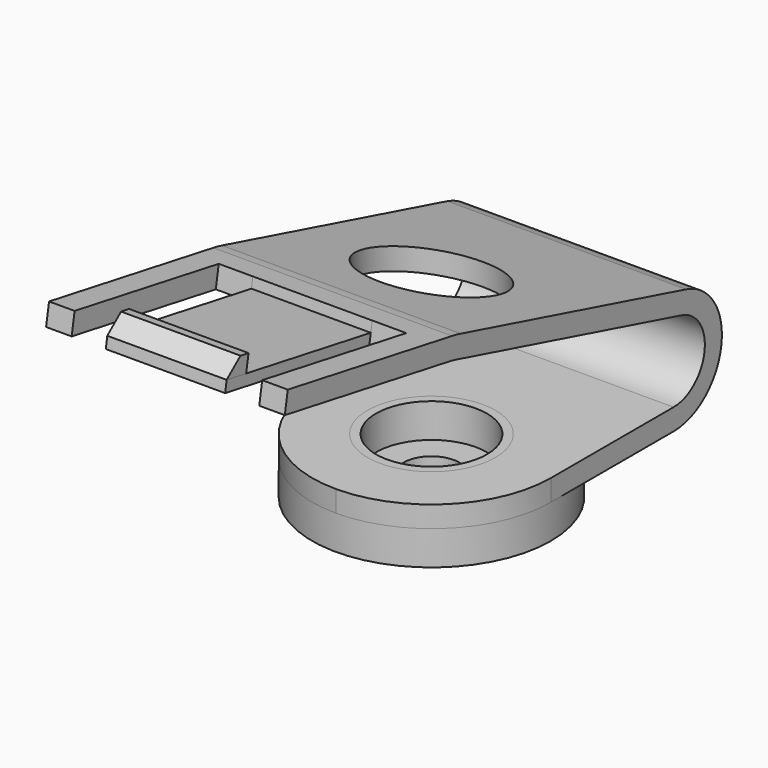
from build123d import *
from build123d import SkipClean  # not in build123d's __all__

# Parameters (mm, degrees)
F1_DEPTH    = 28
F2_T1_DEPTH = 28
F2_T3_DEPTH = 31.2745707181
F3_R        = 14
F4_DEPTH    = 4
F6_DEPTH    = 2.5
F7_R        = 3.25
F8_DEPTH    = 31.3042238242
F9_R        = 7.5
F10_DEPTH   = 24.8042238242
F11_R       = 6.5
F12_DEPTH   = 4
F13_W       = 4
F13_H       = 21.4542382136
F14_DEPTH   = 2.5
F15_W       = 14
F15_H       = 21.4542382136
F16_DEPTH   = 1.2
F18_DEPTH   = 14


# Not quite as in the source:
# - a fillet or chamfer that OpenCascade refuses, or shapes differently, is made with other operations: its cross-section is extruded or revolved along the edge and cut away or added


with BuildPart() as f1:
    # F0 (on Right) → F1 (new body)
    with BuildSketch(Plane.YZ):
        with BuildLine():
            Line((0, 0), (-32, 0))
            Line((-32, 0), (-32, -2.5))
            Line((-32, -2.5), (0, -2.5))
            ThreePointArc((0, -2.5), (7.0205462081, 3.6568537819), (1.8327303277, 11.4209689242))
            Line((1.8327303277, 11.4209689242), (-31.8381916428, 20.4430652746))
            Line((-31.8381916428, 20.4430652746), (-56.5658795558, 24.8032238242))
            Line((-56.5658795558, 24.8032238242), (-57, 22.3412044417))
            Line((-57, 22.3412044417), (-32.3798061747, 18))
            Line((-32.3798061747, 18), (1.1856827149, 9.0061543585))
            ThreePointArc((1.1856827149, 9.0061543585), (4.5419340547, 3.9831692624), (0, 0))
        make_face()
    extrude(amount=F1_DEPTH)

    # F2: fillet of radius 15 on 2 edges, made by hand

    # F2_s2 → F2_t1 (join)
    with BuildSketch(Plane.YZ):
        with BuildLine():
            ThreePointArc((-33.0247707009, 18.1137246476), (-32.3828991568, 17.9860484592), (-31.7472076894, 17.8304957467))
            Line((-31.7472076894, 17.8304957467), (-32.3798061747, 18))
            Line((-32.3798061747, 18), (-33.0247707009, 18.1137246476))
        make_face()
    extrude(amount=F2_T1_DEPTH)

    # F2_s4 → F2_t3 (cut)
    with BuildSketch(Plane.YZ.offset(-1.6372853591)):
        with BuildLine():
            ThreePointArc((-31.2055931575, 20.2735610213), (-31.841284625, 20.4291137338), (-32.483156169, 20.5567899222))
            Line((-32.483156169, 20.5567899222), (-31.8381916428, 20.4430652746))
            Line((-31.8381916428, 20.4430652746), (-31.2055931575, 20.2735610213))
        make_face()
    extrude(amount=F2_T3_DEPTH, mode=Mode.SUBTRACT)

    # F3 (on face) → F4 (join)
    with BuildSketch(Plane(origin=(0, 0, -2.5), x_dir=(1, 0, 0), z_dir=(0, 0, -1))):
        with Locations((14, 18)):
            Circle(F3_R)
    extrude(amount=F4_DEPTH)

    # F5 (on face) → F6 (cut, through all)
    with BuildSketch(Plane(origin=(0, 0, -2.5), x_dir=(1, 0, 0), z_dir=(0, 0, -1))):
        with BuildLine():
            ThreePointArc((0, 18), (4.1005050634, 27.8994949366), (14, 32))
            Line((14, 32), (0, 32))
            Line((0, 32), (0, 18))
        make_face()
        with BuildLine():
            Line((28, 18), (28, 32))
            Line((28, 32), (14, 32))
            ThreePointArc((14, 32), (23.8994949366, 27.8994949366), (28, 18))
        make_face()
    with SkipClean():  # cleaning this boolean's faces spoils the solid; the shape is the same uncleaned
        extrude(amount=-F6_DEPTH, mode=Mode.SUBTRACT)

    # F7 (on face) → F8 (cut, through all)
    with BuildSketch(Plane(origin=(0, 0, -6.5), x_dir=(1, 0, 0), z_dir=(0, 0, -1))):
        with Locations((14, 18)):
            Circle(F7_R)
    with SkipClean():  # cleaning this boolean's faces spoils the solid; the shape is the same uncleaned
        extrude(amount=-F8_DEPTH, mode=Mode.SUBTRACT)

    # F9 (on face) → F10 (cut, through all)
    with BuildSketch(Plane.XY):
        with Locations((14, -18)):
            Circle(F9_R)
    with SkipClean():  # cleaning this boolean's faces spoils the solid; the shape is the same uncleaned
        extrude(amount=F10_DEPTH, mode=Mode.SUBTRACT)

    # F11 (on face) → F12 (cut)
    with BuildSketch(Plane.XY):
        with Locations((14, -18)):
            Circle(F11_R)
    with SkipClean():  # cleaning this boolean's faces spoils the solid; the shape is the same uncleaned
        extrude(amount=-F12_DEPTH, mode=Mode.SUBTRACT)

    # F13 (on face) → F14 (cut, through all)
    with BuildSketch(Plane(origin=(0, 2.5359311092, 14.3819799952), x_dir=(1, 0, 0), z_dir=(0, 0.1736481777, 0.984807753))):
        with Locations((23, -49.2864322531)):
            Rectangle(F13_W, F13_H)
        with Locations((5, -49.2864322531)):
            Rectangle(F13_W, F13_H)
    with SkipClean():  # cleaning this boolean's faces spoils the solid; the shape is the same uncleaned
        extrude(amount=-F14_DEPTH, mode=Mode.SUBTRACT)

    # F15 (on face) → F16 (cut)
    with BuildSketch(Plane(origin=(0, 2.5359311092, 14.3819799952), x_dir=(1, 0, 0), z_dir=(0, 0.1736481777, 0.984807753))):
        with Locations((14, -49.2864322531)):
            Rectangle(F15_W, F15_H)
    with SkipClean():  # cleaning this boolean's faces spoils the solid; the shape is the same uncleaned
        extrude(amount=-F16_DEPTH, mode=Mode.SUBTRACT)

    # F17 (on face) → F18 (join, through all)
    with BuildSketch(Plane(origin=(7, 0, 0), x_dir=(0, -1, 0), z_dir=(-1, 0, 0))):
        Polygon((53.5699966888, 25.0873101332), (53.9172930442, 23.1176946272), (56.774257369, 23.6214545206), (54.7517659925, 25.2956879464), align=None)
    with SkipClean():  # cleaning this boolean's faces spoils the solid; the shape is the same uncleaned
        extrude(amount=-F18_DEPTH)


solid = f1.part
